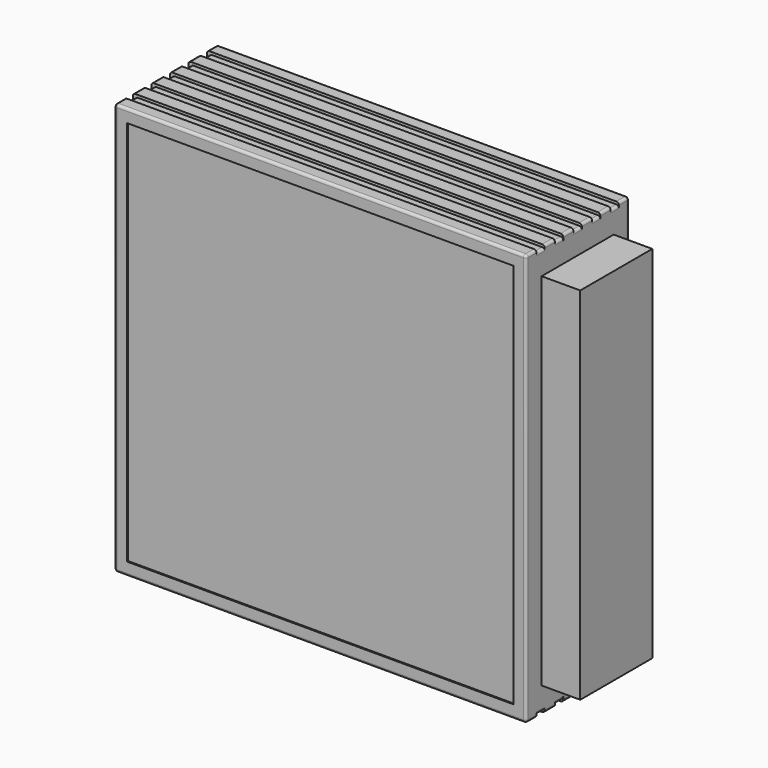
from build123d import *

# Parameters (mm, degrees)
F0_W          = 50
F0_H          = 2720
F1_DEPTH      = 100
F2_W          = 320
F2_H          = 100
F3_DEPTH      = 320
F2_W_2        = 3000
F2_W_3        = 1220
F4_W          = 300
F4_H          = 300
F4_W_2        = 2980
F4_W_3        = 1200
F5_DEPTH      = 100.001
F6_W          = 8
F6_H          = 2
F7_DEPTH      = 4640.001
F8_W          = 2
F8_H          = 8
F9_DEPTH      = 2720.001
F11_W         = 2980
F11_H         = 300
F12_DEPTH     = 98
F11_W_2       = 1200
F11_W_3       = 300
F13_R         = 1.9999
F13_2_R       = 1.9999
F13_3_R       = 1.9999
F13_4_R       = 1.9999
F15_W         = 70
F15_H         = 280
F16_DEPTH     = 30
F17_T1_DEPTH  = 326.0002
F17_T3_DEPTH  = 326.0002
F17_T6_ANGLE  = 90
F17_T8_ANGLE  = 90
F17_T10_ANGLE = 90
F17_T12_ANGLE = 90
F17_T14_ANGLE = 90
F17_T16_ANGLE = 90
F17_T18_ANGLE = 90
F17_T20_ANGLE = 90


# Not quite as in the source:
# - a fillet or chamfer that OpenCascade refuses, or shapes differently, is made with other operations: its cross-section is extruded or revolved along the edge and cut away or added
# - a fillet or chamfer is up to 0.001 mm smaller than in the source, because OpenCascade refuses the exact size


with BuildPart() as f1:
    # F0 (on Front) → F1 (new body)
    with BuildSketch(Plane.XZ):
        with Locations((-1525, -1360)):
            Rectangle(F0_W, F0_H)
    extrude(amount=F1_DEPTH)


with BuildPart() as f1b:
    # F0 (on Front) → F1, piece 2 (new body)
    with BuildSketch(Plane.XZ):
        with Locations((1525, -1360)):
            Rectangle(F0_W, F0_H)
    extrude(amount=F1_DEPTH)


with BuildPart() as f3:
    # F2 (on face) → F3 (new body)
    with BuildSketch(Plane.XY):
        with Locations((-1710, -50)):
            Rectangle(F2_W, F2_H)
    extrude(amount=-F3_DEPTH)


with BuildPart() as f3b:
    # F2 (on face) → F3, piece 2 (new body)
    with BuildSketch(Plane.XY):
        with Locations((0, -50)):
            Rectangle(F2_W_2, F2_H)
    extrude(amount=-F3_DEPTH)


with BuildPart() as f3c:
    # F2 (on face) → F3, piece 3 (new body)
    with BuildSketch(Plane.XY):
        with Locations((2160, -50)):
            Rectangle(F2_W_3, F2_H)
    extrude(amount=-F3_DEPTH)


with BuildPart() as f5_tool:
    # F4 (on face) → F5 (new body, through all)
    with BuildSketch(Plane.XZ.offset(100)):
        with Locations((-1710, -160)):
            Rectangle(F4_W, F4_H)
        with Locations((0, -160)):
            Rectangle(F4_W_2, F4_H)
        with Locations((2160, -160)):
            Rectangle(F4_W_3, F4_H)
    extrude(amount=-F5_DEPTH)


with BuildPart() as f3_1:
    add(f3.part)

    # F5: cut by f5_tool
    add(f5_tool.part, mode=Mode.SUBTRACT)


with BuildPart() as f3b_1:
    add(f3b.part)

    # F5: cut by f5_tool
    add(f5_tool.part, mode=Mode.SUBTRACT)


with BuildPart() as f3c_1:
    add(f3c.part)

    # F5: cut by f5_tool
    add(f5_tool.part, mode=Mode.SUBTRACT)


with BuildPart() as f7_tool:
    # F6 (on face) → F7 (new body, through all)
    with BuildSketch(Plane(origin=(-1870, 0, 0), x_dir=(0, -1, 0), z_dir=(-1, 0, 0))):
        with Locations((14, -1)):
            Rectangle(F6_W, F6_H)
        with Locations((32, -1)):
            Rectangle(F6_W, F6_H)
        with Locations((50, -1)):
            Rectangle(F6_W, F6_H)
        with Locations((68, -1)):
            Rectangle(F6_W, F6_H)
        with Locations((86, -1)):
            Rectangle(F6_W, F6_H)
        with Locations((86, -319)):
            Rectangle(F6_W, F6_H)
        with Locations((68, -319)):
            Rectangle(F6_W, F6_H)
        with Locations((14, -319)):
            Rectangle(F6_W, F6_H)
        with Locations((32, -319)):
            Rectangle(F6_W, F6_H)
        with Locations((50, -319)):
            Rectangle(F6_W, F6_H)
    extrude(amount=-F7_DEPTH)


with BuildPart() as f1_1:
    add(f1.part)

    # F7: cut by f7_tool
    add(f7_tool.part, mode=Mode.SUBTRACT)


with BuildPart() as f1b_1:
    add(f1b.part)

    # F7: cut by f7_tool
    add(f7_tool.part, mode=Mode.SUBTRACT)

    # F13 (radius 2 in the source; OpenCascade refuses exactly that, so slightly less here)
    f13_edges = [f1b_1.edges().sort_by_distance(p)[0] for p in [
        (1525, -90, 0),
        (1525, -100, 0),
        (1525, -72, 0),
        (1525, -82, 0),
        (1525, -54, 0),
        (1525, -64, 0),
        (1525, -36, 0),
        (1525, -46, 0),
        (1525, -18, 0),
        (1525, -28, 0),
        (1525, 0, 0),
        (1525, -10, 0),
    ]]
    fillet(f13_edges, radius=F13_R)


with BuildPart() as f3_2:
    add(f3_1.part)

    # F7: cut by f7_tool
    add(f7_tool.part, mode=Mode.SUBTRACT)


with BuildPart() as f3b_2:
    add(f3b_1.part)

    # F7: cut by f7_tool
    add(f7_tool.part, mode=Mode.SUBTRACT)

    # F13#3 (radius 2 in the source; OpenCascade refuses exactly that, so slightly less here)
    f13_3_edges = [f3b_2.edges().sort_by_distance(p)[0] for p in [
        (1500, -95, 0),
        (1500, -77, 0),
        (1500, -59, 0),
        (1500, -41, 0),
        (1500, -23, 0),
        (1500, -5, 0),
        (1500, -86, -2),
        (1500, -68, -2),
        (1500, -50, -2),
        (1500, -32, -2),
        (1500, -14, -2),
        (1500, -95, -320),
        (1500, -86, -318),
        (1500, -77, -320),
        (1500, -68, -318),
        (1500, -59, -320),
        (1500, -50, -318),
        (1500, -41, -320),
        (1500, -32, -318),
        (1500, -23, -320),
        (1500, -14, -318),
        (1500, -5, -320),
        (-1500, -5, -320),
        (-1500, -23, -320),
        (-1500, -32, -318),
        (-1500, -41, -320),
        (-1500, -50, -318),
        (-1500, -59, -320),
        (-1500, -68, -318),
        (-1500, -77, -320),
        (-1500, -86, -318),
        (-1500, -95, -320),
        (-1500, -14, -318),
        (-1500, -95, 0),
        (-1500, -77, 0),
        (-1500, -59, 0),
        (-1500, -68, -2),
        (-1500, -86, -2),
        (-1500, -50, -2),
        (-1500, -41, 0),
        (-1500, -32, -2),
        (-1500, -23, 0),
        (-1500, -14, -2),
        (-1500, -5, 0),
    ]]
    fillet(f13_3_edges, radius=F13_3_R)


with BuildPart() as f3c_2:
    add(f3c_1.part)

    # F7: cut by f7_tool
    add(f7_tool.part, mode=Mode.SUBTRACT)


with BuildPart() as f9_tool:
    # F8 (on face) → F9 (new body, through all)
    with BuildSketch(Plane.XY):
        with Locations((-1869, -86)):
            Rectangle(F8_W, F8_H)
        with Locations((-1869, -68)):
            Rectangle(F8_W, F8_H)
        with Locations((-1869, -50)):
            Rectangle(F8_W, F8_H)
        with Locations((-1869, -32)):
            Rectangle(F8_W, F8_H)
        with Locations((-1869, -14)):
            Rectangle(F8_W, F8_H)
        with Locations((1869, -68)):
            Rectangle(F8_W, F8_H)
        with Locations((1869, -32)):
            Rectangle(F8_W, F8_H)
        with Locations((1869, -86)):
            Rectangle(F8_W, F8_H)
        with Locations((1869, -50)):
            Rectangle(F8_W, F8_H)
        with Locations((1869, -14)):
            Rectangle(F8_W, F8_H)
    extrude(amount=-F9_DEPTH)


with BuildPart() as f3_3:
    add(f3_2.part)

    # F9: cut by f9_tool
    add(f9_tool.part, mode=Mode.SUBTRACT)

    # F13#2 (radius 2 in the source; OpenCascade refuses exactly that, so slightly less here)
    f13_2_edges = [f3_3.edges().sort_by_distance(p)[0] for p in [
        (-1550, -5, -320),
        (-1550, -14, -318),
        (-1550, -23, -320),
        (-1550, -32, -318),
        (-1550, -41, -320),
        (-1550, -50, -318),
        (-1550, -59, -320),
        (-1550, -68, -318),
        (-1550, -77, -320),
        (-1550, -86, -318),
        (-1550, -95, -320),
        (-1870, -95, -320),
        (-1868, -86, -318),
        (-1870, -77, -320),
        (-1868, -68, -318),
        (-1870, -59, -320),
        (-1868, -50, -318),
        (-1870, -41, -320),
        (-1868, -32, -318),
        (-1870, -23, -320),
        (-1868, -14, -318),
        (-1870, -5, -320),
        (-1870, -95, 0),
        (-1868, -86, -2),
        (-1870, -77, 0),
        (-1868, -68, -2),
        (-1870, -59, 0),
        (-1868, -50, -2),
        (-1870, -41, 0),
        (-1868, -32, -2),
        (-1870, -23, 0),
        (-1868, -14, -2),
        (-1870, -5, 0),
        (-1550, -95, 0),
        (-1550, -77, 0),
        (-1550, -59, 0),
        (-1550, -41, 0),
        (-1550, -23, 0),
        (-1550, -5, 0),
        (-1550, -14, -2),
        (-1550, -32, -2),
        (-1550, -50, -2),
        (-1550, -68, -2),
        (-1550, -86, -2),
    ]]
    fillet(f13_2_edges, radius=F13_2_R)

    # F17: fillet of radius 2 on 16 edges, made by hand

    # F17_s2 → F17_t1 (cut)
    with BuildSketch(Plane.YZ.offset(-1873.0001)):
        with BuildLine():
            ThreePointArc((-100, -2), (-99.4142135624, -0.5857864376), (-98, 0))
            Line((-98, 0), (-98, 0.04))
            Line((-98, 0.04), (-100.04, 0.04))
            Line((-100.04, 0.04), (-100.04, -2))
            Line((-100.04, -2), (-100, -2))
        make_face()
        with BuildLine():
            ThreePointArc((0, -2), (-0.5857864376, -0.5857864376), (-2, 0))
            Line((-2, 0), (-2, 0.04))
            Line((-2, 0.04), (0.04, 0.04))
            Line((0.04, 0.04), (0.04, -2))
            Line((0.04, -2), (0, -2))
        make_face()
        with BuildLine():
            ThreePointArc((-100, -318), (-99.4142135624, -319.4142135624), (-98, -320))
            Line((-98, -320), (-98, -320.04))
            Line((-98, -320.04), (-100.04, -320.04))
            Line((-100.04, -320.04), (-100.04, -318))
            Line((-100.04, -318), (-100, -318))
        make_face()
        with BuildLine():
            ThreePointArc((0, -318), (-0.5857864376, -319.4142135624), (-2, -320))
            Line((-2, -320), (-2, -320.04))
            Line((-2, -320.04), (0.04, -320.04))
            Line((0.04, -320.04), (0.04, -318))
            Line((0.04, -318), (0, -318))
        make_face()
    extrude(amount=F17_T1_DEPTH, mode=Mode.SUBTRACT)

    # F17_s4 → F17_t3 (cut)
    with BuildSketch(Plane.XY.offset(-323.0001)):
        with BuildLine():
            ThreePointArc((-1868, -100), (-1869.4142135624, -99.4142135624), (-1870, -98))
            Line((-1870, -98), (-1870.04, -98))
            Line((-1870.04, -98), (-1870.04, -100.04))
            Line((-1870.04, -100.04), (-1868, -100.04))
            Line((-1868, -100.04), (-1868, -100))
        make_face()
        with BuildLine():
            ThreePointArc((-1552, -100), (-1550.5857864376, -99.4142135624), (-1550, -98))
            Line((-1550, -98), (-1549.96, -98))
            Line((-1549.96, -98), (-1549.96, -100.04))
            Line((-1549.96, -100.04), (-1552, -100.04))
            Line((-1552, -100.04), (-1552, -100))
        make_face()
        with BuildLine():
            ThreePointArc((-1550, -2), (-1550.5857864376, -0.5857864376), (-1552, 0))
            Line((-1552, 0), (-1552, 0.04))
            Line((-1552, 0.04), (-1549.96, 0.04))
            Line((-1549.96, 0.04), (-1549.96, -2))
            Line((-1549.96, -2), (-1550, -2))
        make_face()
        with BuildLine():
            ThreePointArc((-1868, 0), (-1869.4142135624, -0.5857864376), (-1870, -2))
            Line((-1870, -2), (-1870.04, -2))
            Line((-1870.04, -2), (-1870.04, 0.04))
            Line((-1870.04, 0.04), (-1868, 0.04))
            Line((-1868, 0.04), (-1868, 0))
        make_face()
    extrude(amount=F17_T3_DEPTH, mode=Mode.SUBTRACT)

    # F17_s5 → F17_t6 (revolve, cut)
    with BuildSketch(Plane.YZ.offset(-1868.0001)):
        with BuildLine():
            ThreePointArc((-99.9999999975, -1.9999), (-99.4141782066, -0.5857510827), (-98, 0))
            Line((-98, 0), (-98, 0.04))
            Line((-98, 0.04), (-100.04, 0.04))
            Line((-100.04, 0.04), (-100.04, -1.9999))
            Line((-100.04, -1.9999), (-99.9999999975, -1.9999))
        make_face()
    revolve(axis=Axis((-1868.0001, -100, -1.9999), (0, -1, 0)), revolution_arc=F17_T6_ANGLE, mode=Mode.SUBTRACT)

    # F17_s7 → F17_t8 (revolve, cut)
    with BuildSketch(Plane.YZ.offset(-1868.0001)):
        with BuildLine():
            ThreePointArc((-99.9999999975, -318.0001), (-99.4141782066, -319.4142489173), (-98, -320))
            Line((-98, -320), (-98, -320.04))
            Line((-98, -320.04), (-100.04, -320.04))
            Line((-100.04, -320.04), (-100.04, -318.0001))
            Line((-100.04, -318.0001), (-99.9999999975, -318.0001))
        make_face()
    revolve(axis=Axis((-1868.0001, -100, -318.0001), (0, 1, 0)), revolution_arc=F17_T8_ANGLE, mode=Mode.SUBTRACT)

    # F17_s9 → F17_t10 (revolve, cut)
    with BuildSketch(Plane.XY.offset(-1.9999)):
        with BuildLine():
            ThreePointArc((-1551.9999, -99.9999999975), (-1550.5857510827, -99.4141782066), (-1550, -98))
            Line((-1550, -98), (-1549.96, -98))
            Line((-1549.96, -98), (-1549.96, -100.04))
            Line((-1549.96, -100.04), (-1551.9999, -100.04))
            Line((-1551.9999, -100.04), (-1551.9999, -99.9999999975))
        make_face()
    revolve(axis=Axis((-1551.9999, -100, -1.9999), (0, -1, 0)), revolution_arc=F17_T10_ANGLE, mode=Mode.SUBTRACT)

    # F17_s11 → F17_t12 (revolve, cut)
    with BuildSketch(Plane.XY.offset(-318.0001)):
        with BuildLine():
            ThreePointArc((-1551.9999, -99.9999999975), (-1550.5857510827, -99.4141782066), (-1550, -98))
            Line((-1550, -98), (-1549.96, -98))
            Line((-1549.96, -98), (-1549.96, -100.04))
            Line((-1549.96, -100.04), (-1551.9999, -100.04))
            Line((-1551.9999, -100.04), (-1551.9999, -99.9999999975))
        make_face()
    revolve(axis=Axis((-1551.9999, -100, -318.0001), (0, 1, 0)), revolution_arc=F17_T12_ANGLE, mode=Mode.SUBTRACT)

    # F17_s13 → F17_t14 (revolve, cut)
    with BuildSketch(Plane.YZ.offset(-1551.9999)):
        with BuildLine():
            ThreePointArc((-2, 0), (-0.5858217934, -0.5857510827), (-2.5e-09, -1.9999))
            Line((-2.5e-09, -1.9999), (0.04, -1.9999))
            Line((0.04, -1.9999), (0.04, 0.04))
            Line((0.04, 0.04), (-2, 0.04))
            Line((-2, 0.04), (-2, 0))
        make_face()
    revolve(axis=Axis((-1551.9999, 0, -1.9999), (0, 1, 0)), revolution_arc=F17_T14_ANGLE, mode=Mode.SUBTRACT)

    # F17_s15 → F17_t16 (revolve, cut)
    with BuildSketch(Plane.YZ.offset(-1551.9999)):
        with BuildLine():
            ThreePointArc((-2.5e-09, -318.0001), (-0.5858217934, -319.4142489173), (-2, -320))
            Line((-2, -320), (-2, -320.04))
            Line((-2, -320.04), (0.04, -320.04))
            Line((0.04, -320.04), (0.04, -318.0001))
            Line((0.04, -318.0001), (-2.5e-09, -318.0001))
        make_face()
    revolve(axis=Axis((-1551.9999, 0, -318.0001), (0, -1, 0)), revolution_arc=F17_T16_ANGLE, mode=Mode.SUBTRACT)

    # F17_s17 → F17_t18 (revolve, cut)
    with BuildSketch(Plane.XY.offset(-1.9999)):
        with BuildLine():
            ThreePointArc((-1868.0001, -2.5e-09), (-1869.4142489173, -0.5858217934), (-1870, -2))
            Line((-1870, -2), (-1870.04, -2))
            Line((-1870.04, -2), (-1870.04, 0.04))
            Line((-1870.04, 0.04), (-1868.0001, 0.04))
            Line((-1868.0001, 0.04), (-1868.0001, -2.5e-09))
        make_face()
    revolve(axis=Axis((-1868.0001, 0, -1.9999), (0, 1, 0)), revolution_arc=F17_T18_ANGLE, mode=Mode.SUBTRACT)

    # F17_s19 → F17_t20 (revolve, cut)
    with BuildSketch(Plane.XY.offset(-318.0001)):
        with BuildLine():
            ThreePointArc((-1868.0001, -2.5e-09), (-1869.4142489173, -0.5858217934), (-1870, -2))
            Line((-1870, -2), (-1870.04, -2))
            Line((-1870.04, -2), (-1870.04, 0.04))
            Line((-1870.04, 0.04), (-1868.0001, 0.04))
            Line((-1868.0001, 0.04), (-1868.0001, -2.5e-09))
        make_face()
    revolve(axis=Axis((-1868.0001, 0, -318.0001), (0, -1, 0)), revolution_arc=F17_T20_ANGLE, mode=Mode.SUBTRACT)


with BuildPart() as f3c_3:
    add(f3c_2.part)

    # F9: cut by f9_tool
    add(f9_tool.part, mode=Mode.SUBTRACT)

    # F13#4 (radius 2 in the source; OpenCascade refuses exactly that, so slightly less here)
    f13_4_edges = [f3c_3.edges().sort_by_distance(p)[0] for p in [
        (2770, -5, 0),
        (2770, -23, 0),
        (2770, -41, 0),
        (2770, -59, 0),
        (2770, -77, 0),
        (2770, -95, 0),
        (1868, -86, -2),
        (1868, -68, -2),
        (1868, -50, -2),
        (1868, -32, -2),
        (1868, -14, -2),
        (1550, -5, 0),
        (1550, -23, 0),
        (1550, -41, 0),
        (1550, -59, 0),
        (1550, -95, 0),
        (1550, -77, 0),
        (1550, -86, -2),
        (1550, -68, -2),
        (1550, -50, -2),
        (1550, -32, -2),
        (1550, -14, -2),
        (2770, -5, -320),
        (1868, -14, -318),
        (2770, -23, -320),
        (1868, -32, -318),
        (2770, -41, -320),
        (1868, -50, -318),
        (2770, -59, -320),
        (1868, -68, -318),
        (2770, -77, -320),
        (1868, -86, -318),
        (2770, -95, -320),
        (1550, -5, -320),
        (1550, -14, -318),
        (1550, -23, -320),
        (1550, -32, -318),
        (1550, -41, -320),
        (1550, -50, -318),
        (1550, -59, -320),
        (1550, -68, -318),
        (1550, -77, -320),
        (1550, -86, -318),
        (1550, -95, -320),
    ]]
    fillet(f13_4_edges, radius=F13_4_R)


with BuildPart() as f12:
    # F11 (on offset) → F12 (new body, through all)
    with BuildSketch(Plane(origin=(0, -1, 0), x_dir=(-1, 0, 0), z_dir=(0, 1, 0))):
        with Locations((0, -160)):
            Rectangle(F11_W, F11_H)
    extrude(amount=-F12_DEPTH)


with BuildPart() as f12b:
    # F11 (on offset) → F12, piece 2 (new body, through all)
    with BuildSketch(Plane(origin=(0, -1, 0), x_dir=(-1, 0, 0), z_dir=(0, 1, 0))):
        with Locations((-2160, -160)):
            Rectangle(F11_W_2, F11_H)
    extrude(amount=-F12_DEPTH)


with BuildPart() as f12c:
    # F11 (on offset) → F12, piece 3 (new body, through all)
    with BuildSketch(Plane(origin=(0, -1, 0), x_dir=(-1, 0, 0), z_dir=(0, 1, 0))):
        with Locations((1710, -160)):
            Rectangle(F11_W_3, F11_H)
    extrude(amount=-F12_DEPTH)


with BuildPart() as f16:
    # F15 (on face) → F16 (new body)
    with BuildSketch(Plane.YZ.offset(-1550)):
        with Locations((-50, -160)):
            Rectangle(F15_W, F15_H)
    extrude(amount=F16_DEPTH)


solid = Compound([f3_3.part, f12c.part, f16.part])
